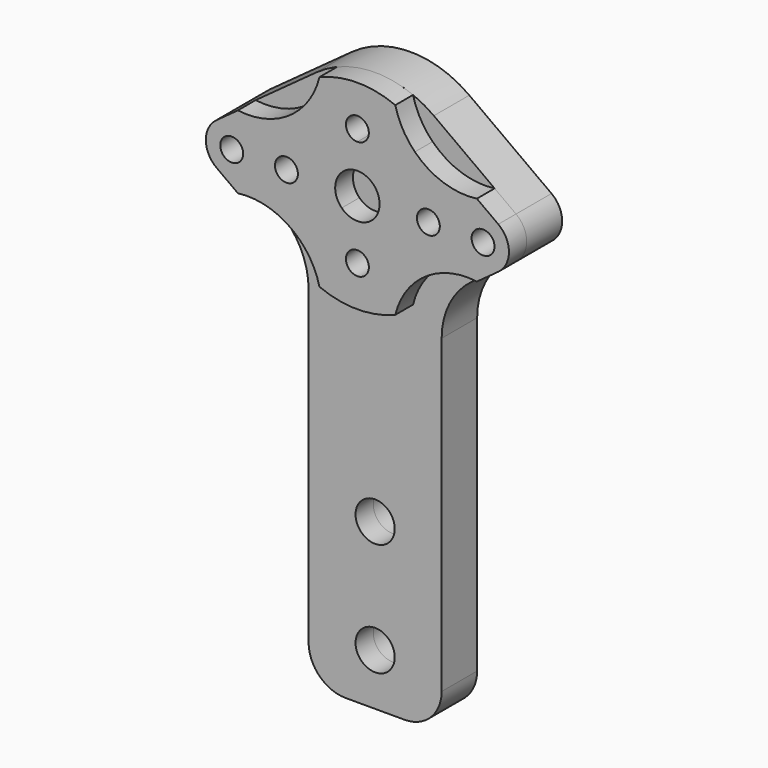
from build123d import *

# Parameters (mm, degrees)
F0_R     = 2.65
F0_R_2   = 1.55
F1_DEPTH = 3
F2_START = 3
F2_DEPTH = 3
F3_R     = 10
F4_R     = 5
F6_DEPTH = 25


with BuildPart() as f1:
    # F0 (on Front) → F1 (new body, symmetric)
    with BuildSketch(Plane.XZ):
        with BuildLine():
            Line((9, -10.147131896), (7.9411764706, -10.917312685))
            ThreePointArc((7.9411764706, -10.917312685), (0, -13.5), (-7.9411764706, -10.917312685))
            Line((-7.9411764706, -10.917312685), (-9, -10.147131896))
            Line((-9, -10.147131896), (-9, -62.3))
            Line((-9, -62.3), (9, -62.3))
            Line((9, -62.3), (9, -10.147131896))
        make_face()
        with Locations((0, -55.3)):
            Circle(F0_R, mode=Mode.SUBTRACT)
        with Locations((0, -40)):
            Circle(F0_R, mode=Mode.SUBTRACT)
        with BuildLine():
            ThreePointArc((7.9411764706, 10.917312685), (12.0302926472, 6.1255251876), (13.5, 0))
            ThreePointArc((13.5, 0), (12.0302926472, -6.1255251876), (7.9411764706, -10.917312685))
            Line((7.9411764706, -10.917312685), (9, -10.147131896))
            Line((9, -10.147131896), (19.0588235294, -2.8304143998))
            ThreePointArc((19.0588235294, -2.8304143998), (20.5, 0), (19.0588235294, 2.8304143998))
            Line((19.0588235294, 2.8304143998), (7.9411764706, 10.917312685))
        make_face()
        with BuildLine():
            ThreePointArc((18.55, 0), (17, -1.55), (15.45, 0))
            ThreePointArc((15.45, 0), (17, 1.55), (18.55, 0))
        make_face(mode=Mode.SUBTRACT)
        with BuildLine():
            ThreePointArc((7.9411764706, -10.917312685), (12.0302926472, -6.1255251876), (13.5, 0))
            Line((13.5, 0), (12.55, 0))
            ThreePointArc((12.55, 0), (9.6, -2.95), (6.65, 0))
            Line((6.65, 0), (0, 0))
            Line((0, 0), (-6.65, 0))
            ThreePointArc((-6.65, 0), (-9.6, -2.95), (-12.55, 0))
            Line((-12.55, 0), (-13.5, 0))
            ThreePointArc((-13.5, 0), (-12.0302926472, -6.1255251876), (-7.9411764706, -10.917312685))
            ThreePointArc((-7.9411764706, -10.917312685), (0, -13.5), (7.9411764706, -10.917312685))
        make_face()
        with BuildLine():
            ThreePointArc((2.95, -8), (-2.0859650045, -10.0859650045), (0, -5.05))
            ThreePointArc((0, -5.05), (2.0859650045, -5.9140349955), (2.95, -8))
        make_face(mode=Mode.SUBTRACT)
        with BuildLine():
            Line((12.55, 0), (13.5, 0))
            ThreePointArc((13.5, 0), (12.0302926472, 6.1255251876), (7.9411764706, 10.917312685))
            ThreePointArc((7.9411764706, 10.917312685), (0, 13.5), (-7.9411764706, 10.917312685))
            ThreePointArc((-7.9411764706, 10.917312685), (-12.0302926472, 6.1255251876), (-13.5, 0))
            Line((-13.5, 0), (-12.55, 0))
            ThreePointArc((-12.55, 0), (-9.6, 2.95), (-6.65, 0))
            Line((-6.65, 0), (0, 0))
            Line((0, 0), (6.65, 0))
            ThreePointArc((6.65, 0), (9.6, 2.95), (12.55, 0))
        make_face()
        with BuildLine():
            ThreePointArc((2.95, 8), (2.0859650045, 5.9140349955), (0, 5.05))
            ThreePointArc((0, 5.05), (-2.0859650045, 10.0859650045), (2.95, 8))
        make_face(mode=Mode.SUBTRACT)
        with BuildLine():
            ThreePointArc((-13.5, 0), (-12.0302926472, 6.1255251876), (-7.9411764706, 10.917312685))
            Line((-7.9411764706, 10.917312685), (-19.0588235294, 2.8304143998))
            ThreePointArc((-19.0588235294, 2.8304143998), (-20.5, 0), (-19.0588235294, -2.8304143998))
            Line((-19.0588235294, -2.8304143998), (-9, -10.147131896))
            Line((-9, -10.147131896), (-7.9411764706, -10.917312685))
            ThreePointArc((-7.9411764706, -10.917312685), (-12.0302926472, -6.1255251876), (-13.5, 0))
        make_face()
        with Locations((-17, 0)):
            Circle(F0_R_2, mode=Mode.SUBTRACT)
    extrude(amount=F1_DEPTH, both=True)

    # F3
    f3_edges = [f1.edges().sort_by_distance(p)[0] for p in [
        (9, 0, -10.147132),
        (-9, 0, -10.147132),
    ]]
    fillet(f3_edges, radius=F3_R)

    # F4
    f4_edges = [f1.edges().sort_by_distance(p)[0] for p in [
        (9, 0, -62.3),
        (-9, 0, -62.3),
    ]]
    fillet(f4_edges, radius=F4_R)


with BuildPart() as f2:
    # F0 (on Front) → F2 (new body)
    with BuildSketch(Plane.XZ.offset(F2_START)):
        with BuildLine():
            ThreePointArc((-13.5, 0), (-12.0302926472, 6.1255251876), (-7.9411764706, 10.917312685))
            Line((-7.9411764706, 10.917312685), (-19.0588235294, 2.8304143998))
            ThreePointArc((-19.0588235294, 2.8304143998), (-20.5, 0), (-19.0588235294, -2.8304143998))
            Line((-19.0588235294, -2.8304143998), (-9, -10.147131896))
            Line((-9, -10.147131896), (-7.9411764706, -10.917312685))
            ThreePointArc((-7.9411764706, -10.917312685), (-12.0302926472, -6.1255251876), (-13.5, 0))
        make_face()
        with Locations((-17, 0)):
            Circle(F0_R_2, mode=Mode.SUBTRACT)
        with BuildLine():
            Line((12.55, 0), (13.5, 0))
            ThreePointArc((13.5, 0), (12.0302926472, 6.1255251876), (7.9411764706, 10.917312685))
            ThreePointArc((7.9411764706, 10.917312685), (0, 13.5), (-7.9411764706, 10.917312685))
            ThreePointArc((-7.9411764706, 10.917312685), (-12.0302926472, 6.1255251876), (-13.5, 0))
            Line((-13.5, 0), (-12.55, 0))
            ThreePointArc((-12.55, 0), (-9.6, 2.95), (-6.65, 0))
            Line((-6.65, 0), (0, 0))
            Line((0, 0), (6.65, 0))
            ThreePointArc((6.65, 0), (9.6, 2.95), (12.55, 0))
        make_face()
        with BuildLine():
            ThreePointArc((2.95, 8), (2.0859650045, 5.9140349955), (0, 5.05))
            ThreePointArc((0, 5.05), (-2.0859650045, 10.0859650045), (2.95, 8))
        make_face(mode=Mode.SUBTRACT)
        with BuildLine():
            ThreePointArc((7.9411764706, -10.917312685), (12.0302926472, -6.1255251876), (13.5, 0))
            Line((13.5, 0), (12.55, 0))
            ThreePointArc((12.55, 0), (9.6, -2.95), (6.65, 0))
            Line((6.65, 0), (0, 0))
            Line((0, 0), (-6.65, 0))
            ThreePointArc((-6.65, 0), (-9.6, -2.95), (-12.55, 0))
            Line((-12.55, 0), (-13.5, 0))
            ThreePointArc((-13.5, 0), (-12.0302926472, -6.1255251876), (-7.9411764706, -10.917312685))
            ThreePointArc((-7.9411764706, -10.917312685), (0, -13.5), (7.9411764706, -10.917312685))
        make_face()
        with BuildLine():
            ThreePointArc((2.95, -8), (-2.0859650045, -10.0859650045), (0, -5.05))
            ThreePointArc((0, -5.05), (2.0859650045, -5.9140349955), (2.95, -8))
        make_face(mode=Mode.SUBTRACT)
        with BuildLine():
            ThreePointArc((-6.65, 0), (-9.6, 2.95), (-12.55, 0))
            Line((-12.55, 0), (-11.15, 0))
            ThreePointArc((-11.15, 0), (-9.6, 1.55), (-8.05, 0))
            Line((-8.05, 0), (-6.65, 0))
        make_face()
        with BuildLine():
            ThreePointArc((2.95, 8), (-2.0859650045, 10.0859650045), (0, 5.05))
            ThreePointArc((0, 5.05), (2.0859650045, 5.9140349955), (2.95, 8))
        make_face()
        with BuildLine():
            ThreePointArc((1.55, 8), (1.0960155108, 6.9039844892), (0, 6.45))
            ThreePointArc((0, 6.45), (-1.0960155108, 9.0960155108), (1.55, 8))
        make_face(mode=Mode.SUBTRACT)
        with BuildLine():
            Line((11.15, 0), (12.55, 0))
            ThreePointArc((12.55, 0), (9.6, 2.95), (6.65, 0))
            Line((6.65, 0), (8.05, 0))
            ThreePointArc((8.05, 0), (9.6, 1.55), (11.15, 0))
        make_face()
        with BuildLine():
            ThreePointArc((6.65, 0), (9.6, -2.95), (12.55, 0))
            Line((12.55, 0), (11.15, 0))
            ThreePointArc((11.15, 0), (9.6, -1.55), (8.05, 0))
            Line((8.05, 0), (6.65, 0))
        make_face()
        with BuildLine():
            Line((-11.15, 0), (-12.55, 0))
            ThreePointArc((-12.55, 0), (-9.6, -2.95), (-6.65, 0))
            Line((-6.65, 0), (-8.05, 0))
            ThreePointArc((-8.05, 0), (-9.6, -1.55), (-11.15, 0))
        make_face()
        with BuildLine():
            ThreePointArc((2.95, -8), (2.0859650045, -5.9140349955), (0, -5.05))
            ThreePointArc((0, -5.05), (-2.0859650045, -10.0859650045), (2.95, -8))
        make_face()
        with BuildLine():
            ThreePointArc((1.55, -8), (-1.0960155108, -9.0960155108), (0, -6.45))
            ThreePointArc((0, -6.45), (1.0960155108, -6.9039844892), (1.55, -8))
        make_face(mode=Mode.SUBTRACT)
        with BuildLine():
            ThreePointArc((7.9411764706, 10.917312685), (12.0302926472, 6.1255251876), (13.5, 0))
            ThreePointArc((13.5, 0), (12.0302926472, -6.1255251876), (7.9411764706, -10.917312685))
            Line((7.9411764706, -10.917312685), (9, -10.147131896))
            Line((9, -10.147131896), (19.0588235294, -2.8304143998))
            ThreePointArc((19.0588235294, -2.8304143998), (20.5, 0), (19.0588235294, 2.8304143998))
            Line((19.0588235294, 2.8304143998), (7.9411764706, 10.917312685))
        make_face()
        with BuildLine():
            ThreePointArc((18.55, 0), (17, -1.55), (15.45, 0))
            ThreePointArc((15.45, 0), (17, 1.55), (18.55, 0))
        make_face(mode=Mode.SUBTRACT)
    extrude(amount=F2_DEPTH)

    # F5 (on face) → F6 (cut)
    with BuildSketch(Plane.XZ.offset(6)):
        with BuildLine():
            ThreePointArc((-7.9411764706, 10.917312685), (-6.5837062936, 11.785788537), (-5.1324214417, 12.4863225228))
            ThreePointArc((-5.1324214417, 12.4863225228), (-5.2207257313, 17.5495510293), (-7.7781745931, 21.9203102168))
            Line((-7.7781745931, 21.9203102168), (-14.8492424049, 14.8492424049))
            Line((-14.8492424049, 14.8492424049), (-9.6640827638, 9.6640827638))
            Line((-9.6640827638, 9.6640827638), (-7.9411764706, 10.917312685))
        make_face()
        with BuildLine():
            ThreePointArc((-21.9203102168, 7.7781745931), (-19.2764451233, 5.8826446058), (-16.1640466618, 4.9360547357))
            Line((-16.1640466618, 4.9360547357), (-9.6640827638, 9.6640827638))
            Line((-9.6640827638, 9.6640827638), (-14.8492424049, 14.8492424049))
            Line((-14.8492424049, 14.8492424049), (-21.9203102168, 7.7781745931))
        make_face()
        with BuildLine():
            ThreePointArc((-16.1640466618, 4.9360547357), (-11.6394053608, 5.3783952332), (-7.7781745931, 7.7781745931))
            Line((-7.7781745931, 7.7781745931), (-9.6640827638, 9.6640827638))
            Line((-9.6640827638, 9.6640827638), (-16.1640466618, 4.9360547357))
        make_face()
        with BuildLine():
            Line((-9.6640827638, 9.6640827638), (-7.7781745931, 7.7781745931))
            ThreePointArc((-7.7781745931, 7.7781745931), (-6.1314464327, 9.9502595118), (-5.1324214417, 12.4863225228))
            ThreePointArc((-5.1324214417, 12.4863225228), (-6.5837062936, 11.785788537), (-7.9411764706, 10.917312685))
            Line((-7.9411764706, 10.917312685), (-9.6640827638, 9.6640827638))
        make_face()
        with BuildLine():
            ThreePointArc((5.1324214417, 12.4863225228), (6.1314464327, 9.9502595118), (7.7781745931, 7.7781745931))
            Line((7.7781745931, 7.7781745931), (9.6640827638, 9.6640827638))
            Line((9.6640827638, 9.6640827638), (7.9411764706, 10.917312685))
            ThreePointArc((7.9411764706, 10.917312685), (6.5837062936, 11.785788537), (5.1324214417, 12.4863225228))
        make_face()
        with BuildLine():
            Line((9.6640827638, 9.6640827638), (16.1640466618, 4.9360547357))
            ThreePointArc((16.1640466618, 4.9360547357), (19.2764451233, 5.8826446058), (21.9203102168, 7.7781745931))
            Line((21.9203102168, 7.7781745931), (14.8492424049, 14.8492424049))
            Line((14.8492424049, 14.8492424049), (9.6640827638, 9.6640827638))
        make_face()
        with BuildLine():
            Line((9.6640827638, 9.6640827638), (7.7781745931, 7.7781745931))
            ThreePointArc((7.7781745931, 7.7781745931), (11.6394053608, 5.3783952332), (16.1640466618, 4.9360547357))
            Line((16.1640466618, 4.9360547357), (9.6640827638, 9.6640827638))
        make_face()
        with BuildLine():
            ThreePointArc((16.1640466618, -4.9360547357), (11.6394053608, -5.3783952332), (7.7781745931, -7.7781745931))
            Line((7.7781745931, -7.7781745931), (9.6640827638, -9.6640827638))
            Line((9.6640827638, -9.6640827638), (16.1640466618, -4.9360547357))
        make_face()
        with BuildLine():
            ThreePointArc((21.9203102168, -7.7781745931), (19.2764451233, -5.8826446058), (16.1640466618, -4.9360547357))
            Line((16.1640466618, -4.9360547357), (9.6640827638, -9.6640827638))
            Line((9.6640827638, -9.6640827638), (14.8492424049, -14.8492424049))
            Line((14.8492424049, -14.8492424049), (21.9203102168, -7.7781745931))
        make_face()
        with BuildLine():
            ThreePointArc((7.9411764706, -10.917312685), (6.5837062936, -11.785788537), (5.1324214417, -12.4863225228))
            ThreePointArc((5.1324214417, -12.4863225228), (5.2207257313, -17.5495510293), (7.7781745931, -21.9203102168))
            Line((7.7781745931, -21.9203102168), (14.8492424049, -14.8492424049))
            Line((14.8492424049, -14.8492424049), (9.6640827638, -9.6640827638))
            Line((9.6640827638, -9.6640827638), (7.9411764706, -10.917312685))
        make_face()
        with BuildLine():
            Line((9.6640827638, -9.6640827638), (7.7781745931, -7.7781745931))
            ThreePointArc((7.7781745931, -7.7781745931), (6.1314464327, -9.9502595118), (5.1324214417, -12.4863225228))
            ThreePointArc((5.1324214417, -12.4863225228), (6.5837062936, -11.785788537), (7.9411764706, -10.917312685))
            Line((7.9411764706, -10.917312685), (9.6640827638, -9.6640827638))
        make_face()
        with BuildLine():
            ThreePointArc((-7.7781745931, -21.9203102168), (-5.2207257313, -17.5495510293), (-5.1324214417, -12.4863225228))
            ThreePointArc((-5.1324214417, -12.4863225228), (-6.5837062936, -11.785788537), (-7.9411764706, -10.917312685))
            Line((-7.9411764706, -10.917312685), (-9.6640827638, -9.6640827638))
            Line((-9.6640827638, -9.6640827638), (-14.8492424049, -14.8492424049))
            Line((-14.8492424049, -14.8492424049), (-7.7781745931, -21.9203102168))
        make_face()
        with BuildLine():
            ThreePointArc((-5.1324214417, -12.4863225228), (-6.1314464327, -9.9502595118), (-7.7781745931, -7.7781745931))
            Line((-7.7781745931, -7.7781745931), (-9.6640827638, -9.6640827638))
            Line((-9.6640827638, -9.6640827638), (-7.9411764706, -10.917312685))
            ThreePointArc((-7.9411764706, -10.917312685), (-6.5837062936, -11.785788537), (-5.1324214417, -12.4863225228))
        make_face()
        with BuildLine():
            Line((-9.6640827638, -9.6640827638), (-7.7781745931, -7.7781745931))
            ThreePointArc((-7.7781745931, -7.7781745931), (-11.6394053608, -5.3783952332), (-16.1640466618, -4.9360547357))
            Line((-16.1640466618, -4.9360547357), (-9.6640827638, -9.6640827638))
        make_face()
        with BuildLine():
            Line((-9.6640827638, -9.6640827638), (-16.1640466618, -4.9360547357))
            ThreePointArc((-16.1640466618, -4.9360547357), (-19.2764451233, -5.8826446058), (-21.9203102168, -7.7781745931))
            Line((-21.9203102168, -7.7781745931), (-14.8492424049, -14.8492424049))
            Line((-14.8492424049, -14.8492424049), (-9.6640827638, -9.6640827638))
        make_face()
        with BuildLine():
            ThreePointArc((7.7781745931, 21.9203102168), (5.2207257313, 17.5495510293), (5.1324214417, 12.4863225228))
            ThreePointArc((5.1324214417, 12.4863225228), (6.5837062936, 11.785788537), (7.9411764706, 10.917312685))
            Line((7.9411764706, 10.917312685), (9.6640827638, 9.6640827638))
            Line((9.6640827638, 9.6640827638), (14.8492424049, 14.8492424049))
            Line((14.8492424049, 14.8492424049), (7.7781745931, 21.9203102168))
        make_face()
        with BuildLine():
            ThreePointArc((2.1213203436, -2.1213203436), (2.7716385975, -1.1480502971), (3, 0))
            ThreePointArc((3, 0), (2.7716385975, 1.1480502971), (2.1213203436, 2.1213203436))
            Line((2.1213203436, 2.1213203436), (0, 0))
            Line((0, 0), (2.1213203436, -2.1213203436))
        make_face()
        with BuildLine():
            Line((0, 0), (2.1213203436, 2.1213203436))
            ThreePointArc((2.1213203436, 2.1213203436), (1.1480502971, 2.7716385975), (0, 3))
            Line((0, 3), (0, 0))
        make_face()
        with BuildLine():
            Line((0, 0), (0, 3))
            ThreePointArc((0, 3), (-1.1480502971, 2.7716385975), (-2.1213203436, 2.1213203436))
            Line((-2.1213203436, 2.1213203436), (0, 0))
        make_face()
        with BuildLine():
            Line((-2.1213203436, -2.1213203436), (0, 0))
            Line((0, 0), (-2.1213203436, 2.1213203436))
            ThreePointArc((-2.1213203436, 2.1213203436), (-3, 0), (-2.1213203436, -2.1213203436))
        make_face()
        with BuildLine():
            ThreePointArc((-2.1213203436, -2.1213203436), (0, -3), (2.1213203436, -2.1213203436))
            Line((2.1213203436, -2.1213203436), (0, 0))
            Line((0, 0), (-2.1213203436, -2.1213203436))
        make_face()
    extrude(amount=-F6_DEPTH, mode=Mode.SUBTRACT)


solid = Compound([f1.part, f2.part])
